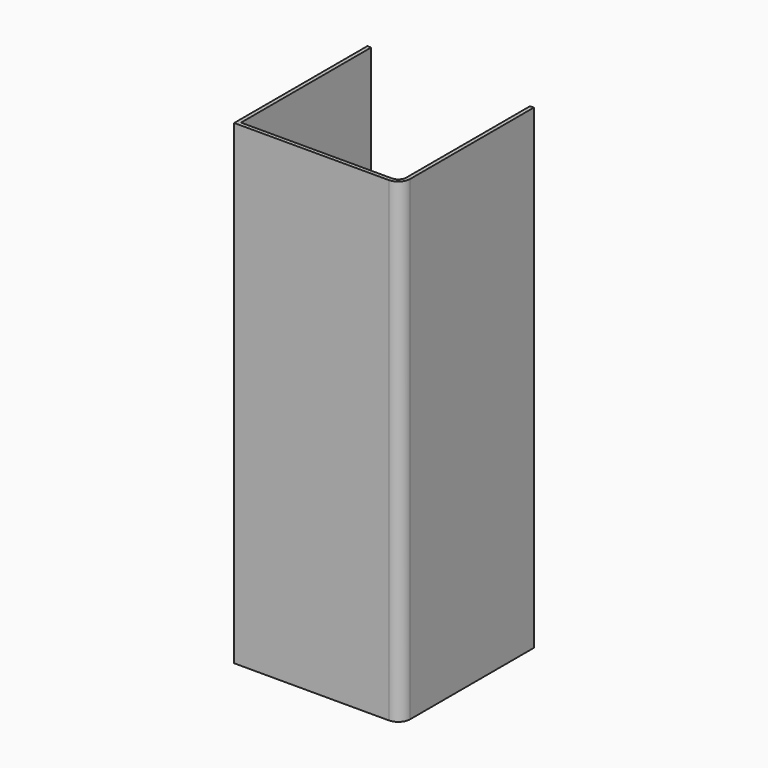
from build123d import *

# Parameters (mm, degrees)
F0_W     = 700
F0_H     = 700
F1_DEPTH = 2000
F2_T     = -16
F3_R     = 50
F4_R     = 34


# Not quite as in the source:
# - a feature names something its author has since deleted; it is built from what else it names


with BuildPart() as f1:
    # F0 (on Top) → F1 (new body)
    with BuildSketch(Plane.XY):
        with Locations((-350, -350)):
            Rectangle(F0_W, F0_H)
    extrude(amount=F1_DEPTH)

    # F2
    f2_openings = [f1.faces().sort_by_distance(p)[0] for p in [
        (-350, 0, 1000),
        (-350, -350, 2000),
        (-350, -350, 0),
    ]]
    offset(amount=F2_T, openings=f2_openings)

    # F3
    f3_edges = [f1.edges().sort_by_distance(p)[0] for p in [
        (0, -700, 1000),
    ]]
    fillet(f3_edges, radius=F3_R)

    # F4
    f4_edges = [f1.edges().sort_by_distance(p)[0] for p in [
        (-16, -684, 1000),
    ]]
    fillet(f4_edges, radius=F4_R)


solid = f1.part
